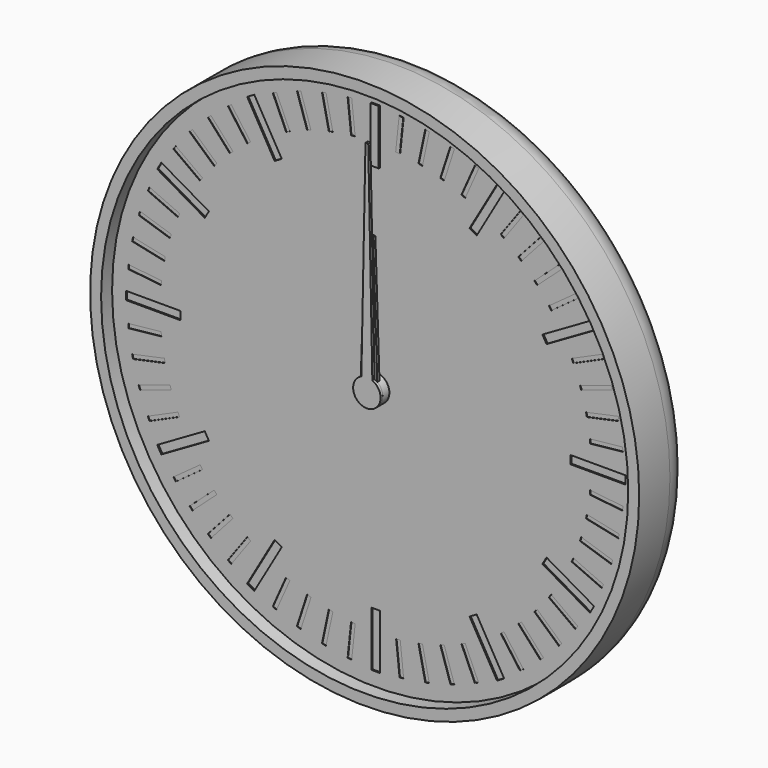
from build123d import *

# Parameters (mm, degrees)
F0_R      = 100
F1_DEPTH  = 24
F2_R      = 10
F3_T      = -4
F4_R      = 5
F4_R_2    = 3
F5_DEPTH  = 2
F6_DEPTH  = 19
F7_DEPTH  = 8
F9_DEPTH  = 4
F11_DEPTH = 4
F12_R     = 5
F12_R_2   = 3
F13_DEPTH = 2
F14_R     = 3
F15_DEPTH = 4
F17_DEPTH = 4
F18_R     = 3
F19_DEPTH = 2
F20_R     = 98
F20_R_2   = 5
F21_DEPTH = 1
F23_R     = 5
F23_R_2   = 3
F24_DEPTH = 2
F25_W     = 3
F25_H     = 20
F25_W_2   = 20
F25_H_2   = 3
F26_DEPTH = 0.5
F27_W     = 1.5
F27_H     = 12
F27_W_2   = 12
F27_H_2   = 1.5
F28_DEPTH = 0.2
F29_DEPTH = 1
F30_DEPTH = 0.4
F31_R     = 5
F31_R_2   = 3
F32_DEPTH = 5
F33_R     = 3
F34_DEPTH = 1
F36_DEPTH = 1


with BuildPart() as f1:
    # F0 (on Front) → F1 (new body)
    with BuildSketch(Plane.XZ):
        Circle(F0_R)
    extrude(amount=F1_DEPTH)

    # F2
    f2_edges = [f1.edges().sort_by_distance(p)[0] for p in [
        (-100, 0, 0),
    ]]
    fillet(f2_edges, radius=F2_R)

    # F3
    f3_openings = [f1.faces().sort_by_distance(p)[0] for p in [
        (0, -24, 0),
    ]]
    offset(amount=F3_T, openings=f3_openings)

    # F4 (on face) → F5 (join)
    with BuildSketch(Plane.XZ.offset(4)):
        Circle(F4_R)
        Circle(F4_R_2, mode=Mode.SUBTRACT)
        with Locations((40, 0)):
            Circle(F4_R)
        with Locations((40, 0)):
            Circle(F4_R_2, mode=Mode.SUBTRACT)
    extrude(amount=F5_DEPTH)


with BuildPart() as f6:
    # F6 (new): a face of the model
    f6_faces = [f1.part.faces().sort_by_distance(p)[0] for p in [
        (0, -4, 0),
    ]]
    extrude(f6_faces, amount=F6_DEPTH)

    # F8 (on face) → F9 (join)
    with BuildSketch(Plane.XZ.offset(6)):
        with BuildLine():
            ThreePointArc((9.2729637667, -1.3794085621), (9.3494561423, -0.6915886375), (9.375, 0))
            ThreePointArc((9.375, 0), (9.3494561423, 0.6915886375), (9.2729637667, 1.3794085621))
            ThreePointArc((9.2729637667, 1.3794085621), (8.9161548403, 2.8970343223), (8.3127812852, 4.3345463782))
            ThreePointArc((8.3127812852, 4.3345463782), (7.5845343223, 5.5104867402), (6.6911892658, 6.566476316))
            ThreePointArc((6.6911892658, 6.566476316), (5.5104867402, 7.5845343223), (4.1773988938, 8.3928519278))
            ThreePointArc((4.1773988938, 8.3928519278), (2.8970343223, 8.9161548403), (1.5536078905, 9.2453733036))
            ThreePointArc((1.5536078905, 9.2453733036), (0, 9.375), (-1.5536078905, 9.2453733036))
            ThreePointArc((-1.5536078905, 9.2453733036), (-2.8970343223, 8.9161548403), (-4.1773988938, 8.3928519278))
            ThreePointArc((-4.1773988938, 8.3928519278), (-5.5104867402, 7.5845343223), (-6.6911892658, 6.566476316))
            ThreePointArc((-6.6911892658, 6.566476316), (-7.5845343223, 5.5104867402), (-8.3127812852, 4.3345463782))
            ThreePointArc((-8.3127812852, 4.3345463782), (-8.9161548403, 2.8970343223), (-9.2729637667, 1.3794085621))
            ThreePointArc((-9.2729637667, 1.3794085621), (-9.375, 0), (-9.2729637667, -1.3794085621))
            ThreePointArc((-9.2729637667, -1.3794085621), (-8.9161548403, -2.8970343223), (-8.3127812852, -4.3345463782))
            ThreePointArc((-8.3127812852, -4.3345463782), (-7.5845343223, -5.5104867402), (-6.6911892658, -6.566476316))
            ThreePointArc((-6.6911892658, -6.566476316), (-5.5104867402, -7.5845343223), (-4.1773988938, -8.3928519278))
            ThreePointArc((-4.1773988938, -8.3928519278), (-2.8970343223, -8.9161548403), (-1.5536078905, -9.2453733036))
            ThreePointArc((-1.5536078905, -9.2453733036), (0, -9.375), (1.5536078905, -9.2453733036))
            ThreePointArc((1.5536078905, -9.2453733036), (2.8970343223, -8.9161548403), (4.1773988938, -8.3928519278))
            ThreePointArc((4.1773988938, -8.3928519278), (5.5104867402, -7.5845343223), (6.6911892658, -6.566476316))
            ThreePointArc((6.6911892658, -6.566476316), (7.5845343223, -5.5104867402), (8.3127812852, -4.3345463782))
            ThreePointArc((8.3127812852, -4.3345463782), (8.9161548403, -2.8970343223), (9.2729637667, -1.3794085621))
        make_face()
        with BuildLine():
            ThreePointArc((8.3127812852, 4.3345463782), (8.9161548403, 2.8970343223), (9.2729637667, 1.3794085621))
            Line((9.2729637667, 1.3794085621), (11.1823199426, 2.3946312492))
            Line((11.1823199426, 2.3946312492), (10.8182678729, 3.515068311))
            Line((10.8182678729, 3.515068311), (10.4542158031, 4.6355053728))
            Line((10.4542158031, 4.6355053728), (8.3127812852, 4.3345463782))
        make_face()
        with BuildLine():
            Line((11.1823199426, -2.3946312492), (9.2729637667, -1.3794085621))
            ThreePointArc((9.2729637667, -1.3794085621), (8.9161548403, -2.8970343223), (8.3127812852, -4.3345463782))
            Line((8.3127812852, -4.3345463782), (10.4542158031, -4.6355053728))
            Line((10.4542158031, -4.6355053728), (10.8182678729, -3.515068311))
            Line((10.8182678729, -3.515068311), (11.1823199426, -2.3946312492))
        make_face()
        with BuildLine():
            ThreePointArc((4.1773988938, 8.3928519278), (5.5104867402, 7.5845343223), (6.6911892658, 6.566476316))
            Line((6.6911892658, 6.566476316), (7.6391579371, 8.5101001246))
            Line((7.6391579371, 8.5101001246), (6.6860572448, 9.202568311))
            Line((6.6860572448, 9.202568311), (5.7329565525, 9.8950364974))
            Line((5.7329565525, 9.8950364974), (4.1773988938, 8.3928519278))
        make_face()
        with BuildLine():
            Line((7.6391579371, -8.5101001246), (6.6911892658, -6.566476316))
            ThreePointArc((6.6911892658, -6.566476316), (5.5104867402, -7.5845343223), (4.1773988938, -8.3928519278))
            Line((4.1773988938, -8.3928519278), (5.7329565525, -9.8950364974))
            Line((5.7329565525, -9.8950364974), (6.6860572448, -9.202568311))
            Line((6.6860572448, -9.202568311), (7.6391579371, -8.5101001246))
        make_face()
        with BuildLine():
            ThreePointArc((-1.5536078905, 9.2453733036), (0, 9.375), (1.5536078905, 9.2453733036))
            Line((1.5536078905, 9.2453733036), (1.1780972451, 11.375))
            Line((1.1780972451, 11.375), (0, 11.375))
            Line((0, 11.375), (-1.1780972451, 11.375))
            Line((-1.1780972451, 11.375), (-1.5536078905, 9.2453733036))
        make_face()
        with BuildLine():
            Line((1.1780972451, -11.375), (1.5536078905, -9.2453733036))
            ThreePointArc((1.5536078905, -9.2453733036), (0, -9.375), (-1.5536078905, -9.2453733036))
            Line((-1.5536078905, -9.2453733036), (-1.1780972451, -11.375))
            Line((-1.1780972451, -11.375), (0, -11.375))
            Line((0, -11.375), (1.1780972451, -11.375))
        make_face()
        with BuildLine():
            ThreePointArc((-6.6911892658, 6.566476316), (-5.5104867402, 7.5845343223), (-4.1773988938, 8.3928519278))
            Line((-4.1773988938, 8.3928519278), (-5.7329565525, 9.8950364974))
            Line((-5.7329565525, 9.8950364974), (-6.6860572448, 9.202568311))
            Line((-6.6860572448, 9.202568311), (-7.6391579371, 8.5101001246))
            Line((-7.6391579371, 8.5101001246), (-6.6911892658, 6.566476316))
        make_face()
        with BuildLine():
            Line((-5.7329565525, -9.8950364974), (-4.1773988938, -8.3928519278))
            ThreePointArc((-4.1773988938, -8.3928519278), (-5.5104867402, -7.5845343223), (-6.6911892658, -6.566476316))
            Line((-6.6911892658, -6.566476316), (-7.6391579371, -8.5101001246))
            Line((-7.6391579371, -8.5101001246), (-6.6860572448, -9.202568311))
            Line((-6.6860572448, -9.202568311), (-5.7329565525, -9.8950364974))
        make_face()
        with BuildLine():
            ThreePointArc((-9.2729637667, 1.3794085621), (-8.9161548403, 2.8970343223), (-8.3127812852, 4.3345463782))
            Line((-8.3127812852, 4.3345463782), (-10.4542158031, 4.6355053728))
            Line((-10.4542158031, 4.6355053728), (-10.8182678729, 3.515068311))
            Line((-10.8182678729, 3.515068311), (-11.1823199426, 2.3946312492))
            Line((-11.1823199426, 2.3946312492), (-9.2729637667, 1.3794085621))
        make_face()
        with BuildLine():
            Line((-10.4542158031, -4.6355053728), (-8.3127812852, -4.3345463782))
            ThreePointArc((-8.3127812852, -4.3345463782), (-8.9161548403, -2.8970343223), (-9.2729637667, -1.3794085621))
            Line((-9.2729637667, -1.3794085621), (-11.1823199426, -2.3946312492))
            Line((-11.1823199426, -2.3946312492), (-10.8182678729, -3.515068311))
            Line((-10.8182678729, -3.515068311), (-10.4542158031, -4.6355053728))
        make_face()
    extrude(amount=F9_DEPTH)

    # F35 (on face) → F36 (join)
    with BuildSketch(Plane.XZ.offset(23)):
        with BuildLine():
            ThreePointArc((-2, 4.582575695), (-2.7386127875, -4.1833001327), (5, 0))
            ThreePointArc((5, 0), (4.1833001327, 2.7386127875), (2, 4.582575695))
            ThreePointArc((2, 4.582575695), (0, 5), (-2, 4.582575695))
        make_face()
        with BuildLine():
            ThreePointArc((-2, 4.582575695), (0, 5), (2, 4.582575695))
            Line((2, 4.582575695), (0.5, 80))
            Line((0.5, 80), (0, 80))
            Line((0, 80), (-0.5, 80))
            Line((-0.5, 80), (-2, 4.582575695))
        make_face()
    extrude(amount=-F36_DEPTH)


with BuildPart() as f7:
    # F7 (new): a face of the model
    f7_faces = [f1.part.faces().sort_by_distance(p)[0] for p in [
        (40, -4, 0),
    ]]
    extrude(f7_faces, amount=F7_DEPTH)

    # F10 (on face) → F11 (join)
    with BuildSketch(Plane.XZ.offset(6)):
        with BuildLine():
            ThreePointArc((68.0829066802, -1.5381733945), (68.1144747006, -0.7693746225), (68.125, 0))
            ThreePointArc((68.125, 0), (68.1144747006, 0.7693746225), (68.0829066802, 1.5381733945))
            ThreePointArc((68.0829066802, 1.5381733945), (67.9709283072, 2.9398630294), (67.7890320221, 4.3342039956))
            ThreePointArc((67.7890320221, 4.3342039956), (67.5104012706, 5.8475163042), (67.1494235596, 7.3433252263))
            ThreePointArc((67.1494235596, 7.3433252263), (66.7484645208, 8.6911029668), (66.280643318, 10.0171558733))
            ThreePointArc((66.280643318, 10.0171558733), (65.6934659962, 11.4394680865), (65.0293803521, 12.8275385085))
            ThreePointArc((65.0293803521, 12.8275385085), (64.3569644814, 14.0625), (63.6236643925, 15.2623099717))
            ThreePointArc((63.6236643925, 15.2623099717), (62.7536029668, 16.5314602207), (61.815433119, 17.7511268046))
            ThreePointArc((61.815433119, 17.7511268046), (60.9009482166, 18.8192983038), (59.934217974, 19.8404278876))
            ThreePointArc((59.934217974, 19.8404278876), (58.8192983038, 20.9009482166), (57.6480467764, 21.8989056799))
            ThreePointArc((57.6480467764, 21.8989056799), (56.5314602207, 22.7536029668), (55.3735505752, 23.5514238999))
            ThreePointArc((55.3735505752, 23.5514238999), (54.0625, 24.3569644814), (52.709356105, 25.0895972944))
            ThreePointArc((52.709356105, 25.0895972944), (51.4394680865, 25.6934659962), (50.1409852457, 26.2331096755))
            ThreePointArc((50.1409852457, 26.2331096755), (48.6911029668, 26.7484645208), (47.2152055856, 27.1837531139))
            ThreePointArc((47.2152055856, 27.1837531139), (45.8475163042, 27.5104012706), (44.4652101991, 27.7682826779))
            ThreePointArc((44.4652101991, 27.7682826779), (42.9398630294, 27.9709283072), (41.4057159597, 28.0898484802))
            ThreePointArc((41.4057159597, 28.0898484802), (40, 28.125), (38.5942840403, 28.0898484802))
            ThreePointArc((38.5942840403, 28.0898484802), (37.0601369706, 27.9709283072), (35.5347898009, 27.7682826779))
            ThreePointArc((35.5347898009, 27.7682826779), (34.1524836958, 27.5104012706), (32.7847944144, 27.1837531139))
            ThreePointArc((32.7847944144, 27.1837531139), (31.3088970332, 26.7484645208), (29.8590147543, 26.2331096755))
            ThreePointArc((29.8590147543, 26.2331096755), (28.5605319135, 25.6934659962), (27.290643895, 25.0895972944))
            ThreePointArc((27.290643895, 25.0895972944), (25.9375, 24.3569644814), (24.6264494248, 23.5514238999))
            ThreePointArc((24.6264494248, 23.5514238999), (23.4685397793, 22.7536029668), (22.3519532236, 21.8989056799))
            ThreePointArc((22.3519532236, 21.8989056799), (21.1807016962, 20.9009482166), (20.065782026, 19.8404278876))
            ThreePointArc((20.065782026, 19.8404278876), (19.0990517834, 18.8192983038), (18.184566881, 17.7511268046))
            ThreePointArc((18.184566881, 17.7511268046), (17.2463970332, 16.5314602207), (16.3763356075, 15.2623099717))
            ThreePointArc((16.3763356075, 15.2623099717), (15.6430355186, 14.0625), (14.9706196479, 12.8275385085))
            ThreePointArc((14.9706196479, 12.8275385085), (14.3065340038, 11.4394680865), (13.719356682, 10.0171558733))
            ThreePointArc((13.719356682, 10.0171558733), (13.2515354792, 8.6911029668), (12.8505764404, 7.3433252263))
            ThreePointArc((12.8505764404, 7.3433252263), (12.4895987294, 5.8475163042), (12.2109679779, 4.3342039956))
            ThreePointArc((12.2109679779, 4.3342039956), (12.0290716928, 2.9398630294), (11.9170933198, 1.5381733945))
            ThreePointArc((11.9170933198, 1.5381733945), (11.875, 0), (11.9170933198, -1.5381733945))
            ThreePointArc((11.9170933198, -1.5381733945), (12.0290716928, -2.9398630294), (12.2109679779, -4.3342039956))
            ThreePointArc((12.2109679779, -4.3342039956), (12.4895987294, -5.8475163042), (12.8505764404, -7.3433252263))
            ThreePointArc((12.8505764404, -7.3433252263), (13.2515354792, -8.6911029668), (13.719356682, -10.0171558733))
            ThreePointArc((13.719356682, -10.0171558733), (14.3065340038, -11.4394680865), (14.9706196479, -12.8275385085))
            ThreePointArc((14.9706196479, -12.8275385085), (15.6430355186, -14.0625), (16.3763356075, -15.2623099717))
            ThreePointArc((16.3763356075, -15.2623099717), (17.2463970332, -16.5314602207), (18.184566881, -17.7511268046))
            ThreePointArc((18.184566881, -17.7511268046), (19.0990517834, -18.8192983038), (20.065782026, -19.8404278876))
            ThreePointArc((20.065782026, -19.8404278876), (21.1807016962, -20.9009482166), (22.3519532236, -21.8989056799))
            ThreePointArc((22.3519532236, -21.8989056799), (23.4685397793, -22.7536029668), (24.6264494248, -23.5514238999))
            ThreePointArc((24.6264494248, -23.5514238999), (25.9375, -24.3569644814), (27.290643895, -25.0895972944))
            ThreePointArc((27.290643895, -25.0895972944), (28.5605319135, -25.6934659962), (29.8590147543, -26.2331096755))
            ThreePointArc((29.8590147543, -26.2331096755), (31.3088970332, -26.7484645208), (32.7847944144, -27.1837531139))
            ThreePointArc((32.7847944144, -27.1837531139), (34.1524836958, -27.5104012706), (35.5347898009, -27.7682826779))
            ThreePointArc((35.5347898009, -27.7682826779), (37.0601369706, -27.9709283072), (38.5942840403, -28.0898484802))
            ThreePointArc((38.5942840403, -28.0898484802), (40, -28.125), (41.4057159597, -28.0898484802))
            ThreePointArc((41.4057159597, -28.0898484802), (42.9398630294, -27.9709283072), (44.4652101991, -27.7682826779))
            ThreePointArc((44.4652101991, -27.7682826779), (45.8475163042, -27.5104012706), (47.2152055856, -27.1837531139))
            ThreePointArc((47.2152055856, -27.1837531139), (48.6911029668, -26.7484645208), (50.1409852457, -26.2331096755))
            ThreePointArc((50.1409852457, -26.2331096755), (51.4394680865, -25.6934659962), (52.709356105, -25.0895972944))
            ThreePointArc((52.709356105, -25.0895972944), (54.0625, -24.3569644814), (55.3735505752, -23.5514238999))
            ThreePointArc((55.3735505752, -23.5514238999), (56.5314602207, -22.7536029668), (57.6480467764, -21.8989056799))
            ThreePointArc((57.6480467764, -21.8989056799), (58.8192983038, -20.9009482166), (59.934217974, -19.8404278876))
            ThreePointArc((59.934217974, -19.8404278876), (60.9009482166, -18.8192983038), (61.815433119, -17.7511268046))
            ThreePointArc((61.815433119, -17.7511268046), (62.7536029668, -16.5314602207), (63.6236643925, -15.2623099717))
            ThreePointArc((63.6236643925, -15.2623099717), (64.3569644814, -14.0625), (65.0293803521, -12.8275385085))
            ThreePointArc((65.0293803521, -12.8275385085), (65.6934659962, -11.4394680865), (66.280643318, -10.0171558733))
            ThreePointArc((66.280643318, -10.0171558733), (66.7484645208, -8.6911029668), (67.1494235596, -7.3433252263))
            ThreePointArc((67.1494235596, -7.3433252263), (67.5104012706, -5.8475163042), (67.7890320221, -4.3342039956))
            ThreePointArc((67.7890320221, -4.3342039956), (67.9709283072, -2.9398630294), (68.0829066802, -1.5381733945))
        make_face()
        with BuildLine():
            ThreePointArc((68.0829066802, 1.5381733945), (68.1144747006, 0.7693746225), (68.125, 0))
            ThreePointArc((68.125, 0), (68.1144747006, -0.7693746225), (68.0829066802, -1.5381733945))
            Line((68.0829066802, -1.5381733945), (70.125, -1.1780972451))
            Line((70.125, -1.1780972451), (70.125, 0))
            Line((70.125, 0), (70.125, 1.1780972451))
            Line((70.125, 1.1780972451), (68.0829066802, 1.5381733945))
        make_face()
        with BuildLine():
            ThreePointArc((67.1494235596, 7.3433252263), (67.5104012706, 5.8475163042), (67.7890320221, 4.3342039956))
            Line((67.7890320221, 4.3342039956), (69.7116366623, 5.1109866922))
            Line((69.7116366623, 5.1109866922), (69.4666964721, 6.2633396859))
            Line((69.4666964721, 6.2633396859), (69.2217562819, 7.4156926796))
            Line((69.2217562819, 7.4156926796), (67.1494235596, 7.3433252263))
        make_face()
        with BuildLine():
            Line((69.7116366623, -5.1109866922), (67.7890320221, -4.3342039956))
            ThreePointArc((67.7890320221, -4.3342039956), (67.5104012706, -5.8475163042), (67.1494235596, -7.3433252263))
            Line((67.1494235596, -7.3433252263), (69.2217562819, -7.4156926796))
            Line((69.2217562819, -7.4156926796), (69.4666964721, -6.2633396859))
            Line((69.4666964721, -6.2633396859), (69.7116366623, -5.1109866922))
        make_face()
        with BuildLine():
            ThreePointArc((65.0293803521, 12.8275385085), (65.6934659962, 11.4394680865), (66.280643318, 10.0171558733))
            Line((66.280643318, 10.0171558733), (67.9997322302, 11.1766959857))
            Line((67.9997322302, 11.1766959857), (67.5205569115, 12.2529413727))
            Line((67.5205569115, 12.2529413727), (67.0413815928, 13.3291867596))
            Line((67.0413815928, 13.3291867596), (65.0293803521, 12.8275385085))
        make_face()
        with BuildLine():
            Line((67.9997322302, -11.1766959857), (66.280643318, -10.0171558733))
            ThreePointArc((66.280643318, -10.0171558733), (65.6934659962, -11.4394680865), (65.0293803521, -12.8275385085))
            Line((65.0293803521, -12.8275385085), (67.0413815928, -13.3291867596))
            Line((67.0413815928, -13.3291867596), (67.5205569115, -12.2529413727))
            Line((67.5205569115, -12.2529413727), (67.9997322302, -11.1766959857))
        make_face()
        with BuildLine():
            ThreePointArc((61.815433119, 17.7511268046), (62.7536029668, 16.5314602207), (63.6236643925, 15.2623099717))
            Line((63.6236643925, 15.2623099717), (65.064105142, 16.753930033))
            Line((65.064105142, 16.753930033), (64.3716369555, 17.7070307253))
            Line((64.3716369555, 17.7070307253), (63.6791687691, 18.6601314176))
            Line((63.6791687691, 18.6601314176), (61.815433119, 17.7511268046))
        make_face()
        with BuildLine():
            Line((65.064105142, -16.753930033), (63.6236643925, -15.2623099717))
            ThreePointArc((63.6236643925, -15.2623099717), (62.7536029668, -16.5314602207), (61.815433119, -17.7511268046))
            Line((61.815433119, -17.7511268046), (63.6791687691, -18.6601314176))
            Line((63.6791687691, -18.6601314176), (64.3716369555, -17.7070307253))
            Line((64.3716369555, -17.7070307253), (65.064105142, -16.753930033))
        make_face()
        with BuildLine():
            ThreePointArc((57.6480467764, 21.8989056799), (58.8192983038, 20.9009482166), (59.934217974, 19.8404278876))
            Line((59.934217974, 19.8404278876), (61.0330563882, 21.5989369435))
            Line((61.0330563882, 21.5989369435), (60.1575595166, 22.3872378675))
            Line((60.1575595166, 22.3872378675), (59.282062645, 23.1755387915))
            Line((59.282062645, 23.1755387915), (57.6480467764, 21.8989056799))
        make_face()
        with BuildLine():
            Line((61.0330563882, -21.5989369435), (59.934217974, -19.8404278876))
            ThreePointArc((59.934217974, -19.8404278876), (58.8192983038, -20.9009482166), (57.6480467764, -21.8989056799))
            Line((57.6480467764, -21.8989056799), (59.282062645, -23.1755387915))
            Line((59.282062645, -23.1755387915), (60.1575595166, -22.3872378675))
            Line((60.1575595166, -22.3872378675), (61.0330563882, -21.5989369435))
        make_face()
        with BuildLine():
            ThreePointArc((52.709356105, 25.0895972944), (54.0625, 24.3569644814), (55.3735505752, 23.5514238999))
            Line((55.3735505752, 23.5514238999), (56.0827621424, 25.4999666665))
            Line((56.0827621424, 25.4999666665), (55.0625, 26.089015289))
            Line((55.0625, 26.089015289), (54.0422378576, 26.6780639116))
            Line((54.0422378576, 26.6780639116), (52.709356105, 25.0895972944))
        make_face()
        with BuildLine():
            Line((56.0827621424, -25.4999666665), (55.3735505752, -23.5514238999))
            ThreePointArc((55.3735505752, -23.5514238999), (54.0625, -24.3569644814), (52.709356105, -25.0895972944))
            Line((52.709356105, -25.0895972944), (54.0422378576, -26.6780639116))
            Line((54.0422378576, -26.6780639116), (55.0625, -26.089015289))
            Line((55.0625, -26.089015289), (56.0827621424, -25.4999666665))
        make_face()
        with BuildLine():
            ThreePointArc((47.2152055856, 27.1837531139), (48.6911029668, 26.7484645208), (50.1409852457, 26.2331096755))
            Line((50.1409852457, 26.2331096755), (50.4295740173, 28.2865254836))
            Line((50.4295740173, 28.2865254836), (49.3091369555, 28.6505775534))
            Line((49.3091369555, 28.6505775534), (48.1886998938, 29.0146296232))
            Line((48.1886998938, 29.0146296232), (47.2152055856, 27.1837531139))
        make_face()
        with BuildLine():
            Line((50.4295740173, -28.2865254836), (50.1409852457, -26.2331096755))
            ThreePointArc((50.1409852457, -26.2331096755), (48.6911029668, -26.7484645208), (47.2152055856, -27.1837531139))
            Line((47.2152055856, -27.1837531139), (48.1886998938, -29.0146296232))
            Line((48.1886998938, -29.0146296232), (49.3091369555, -28.6505775534))
            Line((49.3091369555, -28.6505775534), (50.4295740173, -28.2865254836))
        make_face()
        with BuildLine():
            ThreePointArc((41.4057159597, 28.0898484802), (42.9398630294, 27.9709283072), (44.4652101991, 27.7682826779))
            Line((44.4652101991, 27.7682826779), (44.3205634611, 29.8368274034))
            Line((44.3205634611, 29.8368274034), (43.1489199559, 29.959972098))
            Line((43.1489199559, 29.959972098), (41.9772764508, 30.0831167926))
            Line((41.9772764508, 30.0831167926), (41.4057159597, 28.0898484802))
        make_face()
        with BuildLine():
            Line((44.3205634611, -29.8368274034), (44.4652101991, -27.7682826779))
            ThreePointArc((44.4652101991, -27.7682826779), (42.9398630294, -27.9709283072), (41.4057159597, -28.0898484802))
            Line((41.4057159597, -28.0898484802), (41.9772764508, -30.0831167926))
            Line((41.9772764508, -30.0831167926), (43.1489199559, -29.959972098))
            Line((43.1489199559, -29.959972098), (44.3205634611, -29.8368274034))
        make_face()
        with BuildLine():
            ThreePointArc((35.5347898009, 27.7682826779), (37.0601369706, 27.9709283072), (38.5942840403, 28.0898484802))
            Line((38.5942840403, 28.0898484802), (38.0227235492, 30.0831167926))
            Line((38.0227235492, 30.0831167926), (36.8510800441, 29.959972098))
            Line((36.8510800441, 29.959972098), (35.6794365389, 29.8368274034))
            Line((35.6794365389, 29.8368274034), (35.5347898009, 27.7682826779))
        make_face()
        with BuildLine():
            Line((38.0227235492, -30.0831167926), (38.5942840403, -28.0898484802))
            ThreePointArc((38.5942840403, -28.0898484802), (37.0601369706, -27.9709283072), (35.5347898009, -27.7682826779))
            Line((35.5347898009, -27.7682826779), (35.6794365389, -29.8368274034))
            Line((35.6794365389, -29.8368274034), (36.8510800441, -29.959972098))
            Line((36.8510800441, -29.959972098), (38.0227235492, -30.0831167926))
        make_face()
        with BuildLine():
            ThreePointArc((29.8590147543, 26.2331096755), (31.3088970332, 26.7484645208), (32.7847944144, 27.1837531139))
            Line((32.7847944144, 27.1837531139), (31.8113001062, 29.0146296232))
            Line((31.8113001062, 29.0146296232), (30.6908630445, 28.6505775534))
            Line((30.6908630445, 28.6505775534), (29.5704259827, 28.2865254836))
            Line((29.5704259827, 28.2865254836), (29.8590147543, 26.2331096755))
        make_face()
        with BuildLine():
            Line((31.8113001062, -29.0146296232), (32.7847944144, -27.1837531139))
            ThreePointArc((32.7847944144, -27.1837531139), (31.3088970332, -26.7484645208), (29.8590147543, -26.2331096755))
            Line((29.8590147543, -26.2331096755), (29.5704259827, -28.2865254836))
            Line((29.5704259827, -28.2865254836), (30.6908630445, -28.6505775534))
            Line((30.6908630445, -28.6505775534), (31.8113001062, -29.0146296232))
        make_face()
        with BuildLine():
            ThreePointArc((24.6264494248, 23.5514238999), (25.9375, 24.3569644814), (27.290643895, 25.0895972944))
            Line((27.290643895, 25.0895972944), (25.9577621424, 26.6780639116))
            Line((25.9577621424, 26.6780639116), (24.9375, 26.089015289))
            Line((24.9375, 26.089015289), (23.9172378576, 25.4999666665))
            Line((23.9172378576, 25.4999666665), (24.6264494248, 23.5514238999))
        make_face()
        with BuildLine():
            Line((25.9577621424, -26.6780639116), (27.290643895, -25.0895972944))
            ThreePointArc((27.290643895, -25.0895972944), (25.9375, -24.3569644814), (24.6264494248, -23.5514238999))
            Line((24.6264494248, -23.5514238999), (23.9172378576, -25.4999666665))
            Line((23.9172378576, -25.4999666665), (24.9375, -26.089015289))
            Line((24.9375, -26.089015289), (25.9577621424, -26.6780639116))
        make_face()
        with BuildLine():
            ThreePointArc((20.065782026, 19.8404278876), (21.1807016962, 20.9009482166), (22.3519532236, 21.8989056799))
            Line((22.3519532236, 21.8989056799), (20.717937355, 23.1755387915))
            Line((20.717937355, 23.1755387915), (19.8424404834, 22.3872378675))
            Line((19.8424404834, 22.3872378675), (18.9669436118, 21.5989369435))
            Line((18.9669436118, 21.5989369435), (20.065782026, 19.8404278876))
        make_face()
        with BuildLine():
            Line((20.717937355, -23.1755387915), (22.3519532236, -21.8989056799))
            ThreePointArc((22.3519532236, -21.8989056799), (21.1807016962, -20.9009482166), (20.065782026, -19.8404278876))
            Line((20.065782026, -19.8404278876), (18.9669436118, -21.5989369435))
            Line((18.9669436118, -21.5989369435), (19.8424404834, -22.3872378675))
            Line((19.8424404834, -22.3872378675), (20.717937355, -23.1755387915))
        make_face()
        with BuildLine():
            ThreePointArc((16.3763356075, 15.2623099717), (17.2463970332, 16.5314602207), (18.184566881, 17.7511268046))
            Line((18.184566881, 17.7511268046), (16.3208312309, 18.6601314176))
            Line((16.3208312309, 18.6601314176), (15.6283630445, 17.7070307253))
            Line((15.6283630445, 17.7070307253), (14.935894858, 16.753930033))
            Line((14.935894858, 16.753930033), (16.3763356075, 15.2623099717))
        make_face()
        with BuildLine():
            Line((16.3208312309, -18.6601314176), (18.184566881, -17.7511268046))
            ThreePointArc((18.184566881, -17.7511268046), (17.2463970332, -16.5314602207), (16.3763356075, -15.2623099717))
            Line((16.3763356075, -15.2623099717), (14.935894858, -16.753930033))
            Line((14.935894858, -16.753930033), (15.6283630445, -17.7070307253))
            Line((15.6283630445, -17.7070307253), (16.3208312309, -18.6601314176))
        make_face()
        with BuildLine():
            ThreePointArc((13.719356682, 10.0171558733), (14.3065340038, 11.4394680865), (14.9706196479, 12.8275385085))
            Line((14.9706196479, 12.8275385085), (12.9586184072, 13.3291867596))
            Line((12.9586184072, 13.3291867596), (12.4794430885, 12.2529413727))
            Line((12.4794430885, 12.2529413727), (12.0002677698, 11.1766959857))
            Line((12.0002677698, 11.1766959857), (13.719356682, 10.0171558733))
        make_face()
        with BuildLine():
            Line((12.9586184072, -13.3291867596), (14.9706196479, -12.8275385085))
            ThreePointArc((14.9706196479, -12.8275385085), (14.3065340038, -11.4394680865), (13.719356682, -10.0171558733))
            Line((13.719356682, -10.0171558733), (12.0002677698, -11.1766959857))
            Line((12.0002677698, -11.1766959857), (12.4794430885, -12.2529413727))
            Line((12.4794430885, -12.2529413727), (12.9586184072, -13.3291867596))
        make_face()
        with BuildLine():
            ThreePointArc((12.2109679779, 4.3342039956), (12.4895987294, 5.8475163042), (12.8505764404, 7.3433252263))
            Line((12.8505764404, 7.3433252263), (10.7782437181, 7.4156926796))
            Line((10.7782437181, 7.4156926796), (10.5333035279, 6.2633396859))
            Line((10.5333035279, 6.2633396859), (10.2883633377, 5.1109866922))
            Line((10.2883633377, 5.1109866922), (12.2109679779, 4.3342039956))
        make_face()
        with BuildLine():
            Line((10.7782437181, -7.4156926796), (12.8505764404, -7.3433252263))
            ThreePointArc((12.8505764404, -7.3433252263), (12.4895987294, -5.8475163042), (12.2109679779, -4.3342039956))
            Line((12.2109679779, -4.3342039956), (10.2883633377, -5.1109866922))
            Line((10.2883633377, -5.1109866922), (10.5333035279, -6.2633396859))
            Line((10.5333035279, -6.2633396859), (10.7782437181, -7.4156926796))
        make_face()
        with BuildLine():
            ThreePointArc((11.9170933198, -1.5381733945), (11.875, 0), (11.9170933198, 1.5381733945))
            Line((11.9170933198, 1.5381733945), (9.875, 1.1780972451))
            Line((9.875, 1.1780972451), (9.875, 0))
            Line((9.875, 0), (9.875, -1.1780972451))
            Line((9.875, -1.1780972451), (11.9170933198, -1.5381733945))
        make_face()
    extrude(amount=F11_DEPTH)

    # F16 (on face) → F17 (join)
    with BuildSketch(Plane.XZ.offset(12)):
        with BuildLine():
            ThreePointArc((47.4288750323, -1.0304444454), (47.4821976298, -0.5164480894), (47.5, 0))
            ThreePointArc((47.5, 0), (47.4821976298, 0.5164480894), (47.4288750323, 1.0304444454))
            ThreePointArc((47.4288750323, 1.0304444454), (47.1329238722, 2.3176274578), (46.6157661985, 3.532936117))
            ThreePointArc((46.6157661985, 3.532936117), (46.0676274578, 4.4083893922), (45.4044061018, 5.2002302532))
            ThreePointArc((45.4044061018, 5.2002302532), (44.4083893922, 6.0676274578), (43.2756595386, 6.7468551628))
            ThreePointArc((43.2756595386, 6.7468551628), (42.3176274578, 7.1329238722), (41.3156377295, 7.3837048536))
            ThreePointArc((41.3156377295, 7.3837048536), (40, 7.5), (38.6843622705, 7.3837048536))
            ThreePointArc((38.6843622705, 7.3837048536), (37.6823725422, 7.1329238722), (36.7243404614, 6.7468551628))
            ThreePointArc((36.7243404614, 6.7468551628), (35.5916106078, 6.0676274578), (34.5955938982, 5.2002302532))
            ThreePointArc((34.5955938982, 5.2002302532), (33.9323725422, 4.4083893922), (33.3842338015, 3.532936117))
            ThreePointArc((33.3842338015, 3.532936117), (32.8670761278, 2.3176274578), (32.5711249677, 1.0304444454))
            ThreePointArc((32.5711249677, 1.0304444454), (32.5, 0), (32.5711249677, -1.0304444454))
            ThreePointArc((32.5711249677, -1.0304444454), (32.8670761278, -2.3176274578), (33.3842338015, -3.532936117))
            ThreePointArc((33.3842338015, -3.532936117), (33.9323725422, -4.4083893922), (34.5955938982, -5.2002302532))
            ThreePointArc((34.5955938982, -5.2002302532), (35.5916106078, -6.0676274578), (36.7243404614, -6.7468551628))
            ThreePointArc((36.7243404614, -6.7468551628), (37.6823725422, -7.1329238722), (38.6843622705, -7.3837048536))
            ThreePointArc((38.6843622705, -7.3837048536), (40, -7.5), (41.3156377295, -7.3837048536))
            ThreePointArc((41.3156377295, -7.3837048536), (42.3176274578, -7.1329238722), (43.2756595386, -6.7468551628))
            ThreePointArc((43.2756595386, -6.7468551628), (44.4083893922, -6.0676274578), (45.4044061018, -5.2002302532))
            ThreePointArc((45.4044061018, -5.2002302532), (46.0676274578, -4.4083893922), (46.6157661985, -3.532936117))
            ThreePointArc((46.6157661985, -3.532936117), (47.1329238722, -2.3176274578), (47.4288750323, -1.0304444454))
        make_face()
        with BuildLine():
            ThreePointArc((46.6157661985, 3.532936117), (47.1329238722, 2.3176274578), (47.4288750323, 1.0304444454))
            Line((47.4288750323, 1.0304444454), (49.3262785606, 2.0393117971))
            Line((49.3262785606, 2.0393117971), (48.743795249, 3.832011096))
            Line((48.743795249, 3.832011096), (46.6157661985, 3.532936117))
        make_face()
        with BuildLine():
            Line((49.3262785606, -2.0393117971), (47.4288750323, -1.0304444454))
            ThreePointArc((47.4288750323, -1.0304444454), (47.1329238722, -2.3176274578), (46.6157661985, -3.532936117))
            Line((46.6157661985, -3.532936117), (48.743795249, -3.832011096))
            Line((48.743795249, -3.832011096), (49.3262785606, -2.0393117971))
        make_face()
        with BuildLine():
            ThreePointArc((43.2756595386, 6.7468551628), (44.4083893922, 6.0676274578), (45.4044061018, 5.2002302532))
            Line((45.4044061018, 5.2002302532), (46.3464404506, 7.1316868974))
            Line((46.3464404506, 7.1316868974), (44.8214793429, 8.2396359957))
            Line((44.8214793429, 8.2396359957), (43.2756595386, 6.7468551628))
        make_face()
        with BuildLine():
            Line((46.3464404506, -7.1316868974), (45.4044061018, -5.2002302532))
            ThreePointArc((45.4044061018, -5.2002302532), (44.4083893922, -6.0676274578), (43.2756595386, -6.7468551628))
            Line((43.2756595386, -6.7468551628), (44.8214793429, -8.2396359957))
            Line((44.8214793429, -8.2396359957), (46.3464404506, -7.1316868974))
        make_face()
        with BuildLine():
            ThreePointArc((38.6843622705, 7.3837048536), (40, 7.5), (41.3156377295, 7.3837048536))
            Line((41.3156377295, 7.3837048536), (40.9424777961, 9.5))
            Line((40.9424777961, 9.5), (39.0575222039, 9.5))
            Line((39.0575222039, 9.5), (38.6843622705, 7.3837048536))
        make_face()
        with BuildLine():
            Line((40.9424777961, -9.5), (41.3156377295, -7.3837048536))
            ThreePointArc((41.3156377295, -7.3837048536), (40, -7.5), (38.6843622705, -7.3837048536))
            Line((38.6843622705, -7.3837048536), (39.0575222039, -9.5))
            Line((39.0575222039, -9.5), (40.9424777961, -9.5))
        make_face()
        with BuildLine():
            ThreePointArc((34.5955938982, 5.2002302532), (35.5916106078, 6.0676274578), (36.7243404614, 6.7468551628))
            Line((36.7243404614, 6.7468551628), (35.1785206571, 8.2396359957))
            Line((35.1785206571, 8.2396359957), (33.6535595494, 7.1316868974))
            Line((33.6535595494, 7.1316868974), (34.5955938982, 5.2002302532))
        make_face()
        with BuildLine():
            Line((35.1785206571, -8.2396359957), (36.7243404614, -6.7468551628))
            ThreePointArc((36.7243404614, -6.7468551628), (35.5916106078, -6.0676274578), (34.5955938982, -5.2002302532))
            Line((34.5955938982, -5.2002302532), (33.6535595494, -7.1316868974))
            Line((33.6535595494, -7.1316868974), (35.1785206571, -8.2396359957))
        make_face()
        with BuildLine():
            ThreePointArc((32.5711249677, 1.0304444454), (32.8670761278, 2.3176274578), (33.3842338015, 3.532936117))
            Line((33.3842338015, 3.532936117), (31.256204751, 3.832011096))
            Line((31.256204751, 3.832011096), (30.6737214394, 2.0393117971))
            Line((30.6737214394, 2.0393117971), (32.5711249677, 1.0304444454))
        make_face()
        with BuildLine():
            Line((31.256204751, -3.832011096), (33.3842338015, -3.532936117))
            ThreePointArc((33.3842338015, -3.532936117), (32.8670761278, -2.3176274578), (32.5711249677, -1.0304444454))
            Line((32.5711249677, -1.0304444454), (30.6737214394, -2.0393117971))
            Line((30.6737214394, -2.0393117971), (31.256204751, -3.832011096))
        make_face()
    extrude(amount=F17_DEPTH)

    # F18 (on face) → F19 (join)
    with BuildSketch(Plane.XZ.offset(16)):
        with Locations((40, 0)):
            Circle(F18_R)
    extrude(amount=F19_DEPTH)


with BuildPart() as f13:
    # F12 (on face) → F13 (new body)
    with BuildSketch(Plane.XZ.offset(10)):
        Circle(F12_R)
        Circle(F12_R_2, mode=Mode.SUBTRACT)
    extrude(amount=F13_DEPTH)

    # F14 (on face) → F15 (join)
    with BuildSketch(Plane.XZ.offset(12)):
        with BuildLine():
            ThreePointArc((29.9718156995, -1.3001014101), (29.9929530972, -0.6502034357), (30, 0))
            ThreePointArc((30, 0), (29.9929530972, 0.6502034357), (29.9718156995, 1.3001014101))
            ThreePointArc((29.9718156995, 1.3001014101), (29.907520012, 2.3537728718), (29.8061935814, 3.4045299509))
            ThreePointArc((29.8061935814, 3.4045299509), (29.6306502179, 4.6930339512), (29.3994322443, 5.9727199596))
            ThreePointArc((29.3994322443, 5.9727199596), (29.1710976119, 7.0033609157), (28.9066440563, 8.0253304855))
            ThreePointArc((28.9066440563, 8.0253304855), (28.5316954889, 9.2705098312), (28.1031371961, 10.4982703213))
            ThreePointArc((28.1031371961, 10.4982703213), (27.7163859753, 11.480502971), (27.2953170189, 12.448520749))
            ThreePointArc((27.2953170189, 12.448520749), (26.7301957257, 13.6197149922), (26.1148496411, 14.765318426))
            ThreePointArc((26.1148496411, 14.765318426), (25.5792049306, 15.6749569415), (25.0118886885, 16.5651871174))
            ThreePointArc((25.0118886885, 16.5651871174), (24.2705098312, 17.6335575688), (23.4835278178, 18.6687953878))
            ThreePointArc((23.4835278178, 18.6687953878), (22.812178968, 19.4834414499), (22.1125846489, 20.2739636023))
            ThreePointArc((22.1125846489, 20.2739636023), (21.2132034356, 21.2132034356), (20.2739636023, 22.1125846489))
            ThreePointArc((20.2739636023, 22.1125846489), (19.4834414499, 22.812178968), (18.6687953878, 23.4835278178))
            ThreePointArc((18.6687953878, 23.4835278178), (17.6335575688, 24.2705098312), (16.5651871174, 25.0118886885))
            ThreePointArc((16.5651871174, 25.0118886885), (15.6749569415, 25.5792049306), (14.765318426, 26.1148496411))
            ThreePointArc((14.765318426, 26.1148496411), (13.6197149922, 26.7301957257), (12.448520749, 27.2953170189))
            ThreePointArc((12.448520749, 27.2953170189), (11.480502971, 27.7163859753), (10.4982703213, 28.1031371961))
            ThreePointArc((10.4982703213, 28.1031371961), (9.2705098312, 28.5316954889), (8.0253304855, 28.9066440563))
            ThreePointArc((8.0253304855, 28.9066440563), (7.0033609157, 29.1710976119), (5.9727199596, 29.3994322443))
            ThreePointArc((5.9727199596, 29.3994322443), (4.6930339512, 29.6306502179), (3.4045299509, 29.8061935814))
            ThreePointArc((3.4045299509, 29.8061935814), (2.3537728718, 29.907520012), (1.3001014101, 29.9718156995))
            ThreePointArc((1.3001014101, 29.9718156995), (0, 30), (-1.3001014101, 29.9718156995))
            ThreePointArc((-1.3001014101, 29.9718156995), (-2.3537728718, 29.907520012), (-3.4045299509, 29.8061935814))
            ThreePointArc((-3.4045299509, 29.8061935814), (-4.6930339512, 29.6306502179), (-5.9727199596, 29.3994322443))
            ThreePointArc((-5.9727199596, 29.3994322443), (-7.0033609157, 29.1710976119), (-8.0253304855, 28.9066440563))
            ThreePointArc((-8.0253304855, 28.9066440563), (-9.2705098312, 28.5316954889), (-10.4982703213, 28.1031371961))
            ThreePointArc((-10.4982703213, 28.1031371961), (-11.480502971, 27.7163859753), (-12.448520749, 27.2953170189))
            ThreePointArc((-12.448520749, 27.2953170189), (-13.6197149922, 26.7301957257), (-14.765318426, 26.1148496411))
            ThreePointArc((-14.765318426, 26.1148496411), (-15.6749569415, 25.5792049306), (-16.5651871174, 25.0118886885))
            ThreePointArc((-16.5651871174, 25.0118886885), (-17.6335575688, 24.2705098312), (-18.6687953878, 23.4835278178))
            ThreePointArc((-18.6687953878, 23.4835278178), (-19.4834414499, 22.812178968), (-20.2739636023, 22.1125846489))
            ThreePointArc((-20.2739636023, 22.1125846489), (-21.2132034356, 21.2132034356), (-22.1125846489, 20.2739636023))
            ThreePointArc((-22.1125846489, 20.2739636023), (-22.812178968, 19.4834414499), (-23.4835278178, 18.6687953878))
            ThreePointArc((-23.4835278178, 18.6687953878), (-24.2705098312, 17.6335575688), (-25.0118886885, 16.5651871174))
            ThreePointArc((-25.0118886885, 16.5651871174), (-25.5792049306, 15.6749569415), (-26.1148496411, 14.765318426))
            ThreePointArc((-26.1148496411, 14.765318426), (-26.7301957257, 13.6197149922), (-27.2953170189, 12.448520749))
            ThreePointArc((-27.2953170189, 12.448520749), (-27.7163859753, 11.480502971), (-28.1031371961, 10.4982703213))
            ThreePointArc((-28.1031371961, 10.4982703213), (-28.5316954889, 9.2705098312), (-28.9066440563, 8.0253304855))
            ThreePointArc((-28.9066440563, 8.0253304855), (-29.1710976119, 7.0033609157), (-29.3994322443, 5.9727199596))
            ThreePointArc((-29.3994322443, 5.9727199596), (-29.6306502179, 4.6930339512), (-29.8061935814, 3.4045299509))
            ThreePointArc((-29.8061935814, 3.4045299509), (-29.907520012, 2.3537728718), (-29.9718156995, 1.3001014101))
            ThreePointArc((-29.9718156995, 1.3001014101), (-30, 0), (-29.9718156995, -1.3001014101))
            ThreePointArc((-29.9718156995, -1.3001014101), (-29.907520012, -2.3537728718), (-29.8061935814, -3.4045299509))
            ThreePointArc((-29.8061935814, -3.4045299509), (-29.6306502179, -4.6930339512), (-29.3994322443, -5.9727199596))
            ThreePointArc((-29.3994322443, -5.9727199596), (-29.1710976119, -7.0033609157), (-28.9066440563, -8.0253304855))
            ThreePointArc((-28.9066440563, -8.0253304855), (-28.5316954889, -9.2705098312), (-28.1031371961, -10.4982703213))
            ThreePointArc((-28.1031371961, -10.4982703213), (-27.7163859753, -11.480502971), (-27.2953170189, -12.448520749))
            ThreePointArc((-27.2953170189, -12.448520749), (-26.7301957257, -13.6197149922), (-26.1148496411, -14.765318426))
            ThreePointArc((-26.1148496411, -14.765318426), (-25.5792049306, -15.6749569415), (-25.0118886885, -16.5651871174))
            ThreePointArc((-25.0118886885, -16.5651871174), (-24.2705098312, -17.6335575688), (-23.4835278178, -18.6687953878))
            ThreePointArc((-23.4835278178, -18.6687953878), (-22.812178968, -19.4834414499), (-22.1125846489, -20.2739636023))
            ThreePointArc((-22.1125846489, -20.2739636023), (-21.2132034356, -21.2132034356), (-20.2739636023, -22.1125846489))
            ThreePointArc((-20.2739636023, -22.1125846489), (-19.4834414499, -22.812178968), (-18.6687953878, -23.4835278178))
            ThreePointArc((-18.6687953878, -23.4835278178), (-17.6335575688, -24.2705098312), (-16.5651871174, -25.0118886885))
            ThreePointArc((-16.5651871174, -25.0118886885), (-15.6749569415, -25.5792049306), (-14.765318426, -26.1148496411))
            ThreePointArc((-14.765318426, -26.1148496411), (-13.6197149922, -26.7301957257), (-12.448520749, -27.2953170189))
            ThreePointArc((-12.448520749, -27.2953170189), (-11.480502971, -27.7163859753), (-10.4982703213, -28.1031371961))
            ThreePointArc((-10.4982703213, -28.1031371961), (-9.2705098312, -28.5316954889), (-8.0253304855, -28.9066440563))
            ThreePointArc((-8.0253304855, -28.9066440563), (-7.0033609157, -29.1710976119), (-5.9727199596, -29.3994322443))
            ThreePointArc((-5.9727199596, -29.3994322443), (-4.6930339512, -29.6306502179), (-3.4045299509, -29.8061935814))
            ThreePointArc((-3.4045299509, -29.8061935814), (-2.3537728718, -29.907520012), (-1.3001014101, -29.9718156995))
            ThreePointArc((-1.3001014101, -29.9718156995), (0, -30), (1.3001014101, -29.9718156995))
            ThreePointArc((1.3001014101, -29.9718156995), (2.3537728718, -29.907520012), (3.4045299509, -29.8061935814))
            ThreePointArc((3.4045299509, -29.8061935814), (4.6930339512, -29.6306502179), (5.9727199596, -29.3994322443))
            ThreePointArc((5.9727199596, -29.3994322443), (7.0033609157, -29.1710976119), (8.0253304855, -28.9066440563))
            ThreePointArc((8.0253304855, -28.9066440563), (9.2705098312, -28.5316954889), (10.4982703213, -28.1031371961))
            ThreePointArc((10.4982703213, -28.1031371961), (11.480502971, -27.7163859753), (12.448520749, -27.2953170189))
            ThreePointArc((12.448520749, -27.2953170189), (13.6197149922, -26.7301957257), (14.765318426, -26.1148496411))
            ThreePointArc((14.765318426, -26.1148496411), (15.6749569415, -25.5792049306), (16.5651871174, -25.0118886885))
            ThreePointArc((16.5651871174, -25.0118886885), (17.6335575688, -24.2705098312), (18.6687953878, -23.4835278178))
            ThreePointArc((18.6687953878, -23.4835278178), (19.4834414499, -22.812178968), (20.2739636023, -22.1125846489))
            ThreePointArc((20.2739636023, -22.1125846489), (21.2132034356, -21.2132034356), (22.1125846489, -20.2739636023))
            ThreePointArc((22.1125846489, -20.2739636023), (22.812178968, -19.4834414499), (23.4835278178, -18.6687953878))
            ThreePointArc((23.4835278178, -18.6687953878), (24.2705098312, -17.6335575688), (25.0118886885, -16.5651871174))
            ThreePointArc((25.0118886885, -16.5651871174), (25.5792049306, -15.6749569415), (26.1148496411, -14.765318426))
            ThreePointArc((26.1148496411, -14.765318426), (26.7301957257, -13.6197149922), (27.2953170189, -12.448520749))
            ThreePointArc((27.2953170189, -12.448520749), (27.7163859753, -11.480502971), (28.1031371961, -10.4982703213))
            ThreePointArc((28.1031371961, -10.4982703213), (28.5316954889, -9.2705098312), (28.9066440563, -8.0253304855))
            ThreePointArc((28.9066440563, -8.0253304855), (29.1710976119, -7.0033609157), (29.3994322443, -5.9727199596))
            ThreePointArc((29.3994322443, -5.9727199596), (29.6306502179, -4.6930339512), (29.8061935814, -3.4045299509))
            ThreePointArc((29.8061935814, -3.4045299509), (29.907520012, -2.3537728718), (29.9718156995, -1.3001014101))
        make_face()
        Circle(F14_R, mode=Mode.SUBTRACT)
        with BuildLine():
            ThreePointArc((29.9718156995, 1.3001014101), (29.9929530972, 0.6502034357), (30, 0))
            ThreePointArc((30, 0), (29.9929530972, -0.6502034357), (29.9718156995, -1.3001014101))
            Line((29.9718156995, -1.3001014101), (32, -0.9424777961))
            Line((32, -0.9424777961), (32, 0))
            Line((32, 0), (32, 0.9424777961))
            Line((32, 0.9424777961), (29.9718156995, 1.3001014101))
        make_face()
        with BuildLine():
            ThreePointArc((29.3994322443, 5.9727199596), (29.6306502179, 4.6930339512), (29.8061935814, 3.4045299509))
            Line((29.8061935814, 3.4045299509), (31.7534629089, 4.0750285508))
            Line((31.7534629089, 4.0750285508), (31.606026899, 5.0059028813))
            Line((31.606026899, 5.0059028813), (31.4585908892, 5.9367772117))
            Line((31.4585908892, 5.9367772117), (29.3994322443, 5.9727199596))
        make_face()
        with BuildLine():
            Line((31.7534629089, -4.0750285508), (29.8061935814, -3.4045299509))
            ThreePointArc((29.8061935814, -3.4045299509), (29.6306502179, -4.6930339512), (29.3994322443, -5.9727199596))
            Line((29.3994322443, -5.9727199596), (31.4585908892, -5.9367772117))
            Line((31.4585908892, -5.9367772117), (31.606026899, -5.0059028813))
            Line((31.606026899, -5.0059028813), (31.7534629089, -4.0750285508))
        make_face()
        with BuildLine():
            ThreePointArc((28.1031371961, 10.4982703213), (28.5316954889, 9.2705098312), (28.9066440563, 8.0253304855))
            Line((28.9066440563, 8.0253304855), (30.7250501773, 8.9921941706))
            Line((30.7250501773, 8.9921941706), (30.4338085214, 9.88854382))
            Line((30.4338085214, 9.88854382), (30.1425668656, 10.7848934694))
            Line((30.1425668656, 10.7848934694), (28.1031371961, 10.4982703213))
        make_face()
        with BuildLine():
            Line((30.7250501773, -8.9921941706), (28.9066440563, -8.0253304855))
            ThreePointArc((28.9066440563, -8.0253304855), (28.5316954889, -9.2705098312), (28.1031371961, -10.4982703213))
            Line((28.1031371961, -10.4982703213), (30.1425668656, -10.7848934694))
            Line((30.1425668656, -10.7848934694), (30.4338085214, -9.88854382))
            Line((30.4338085214, -9.88854382), (30.7250501773, -8.9921941706))
        make_face()
        with BuildLine():
            ThreePointArc((26.1148496411, 14.765318426), (26.7301957257, 13.6197149922), (27.2953170189, 12.448520749))
            Line((27.2953170189, 12.448520749), (28.9400847397, 13.6879421265))
            Line((28.9400847397, 13.6879421265), (28.512208774, 14.5276959917))
            Line((28.512208774, 14.5276959917), (28.0843328084, 15.3674498569))
            Line((28.0843328084, 15.3674498569), (26.1148496411, 14.765318426))
        make_face()
        with BuildLine():
            Line((28.9400847397, -13.6879421265), (27.2953170189, -12.448520749))
            ThreePointArc((27.2953170189, -12.448520749), (26.7301957257, -13.6197149922), (26.1148496411, -14.765318426))
            Line((26.1148496411, -14.765318426), (28.0843328084, -15.3674498569))
            Line((28.0843328084, -15.3674498569), (28.512208774, -14.5276959917))
            Line((28.512208774, -14.5276959917), (28.9400847397, -13.6879421265))
        make_face()
        with BuildLine():
            ThreePointArc((23.4835278178, 18.6687953878), (24.2705098312, 17.6335575688), (25.0118886885, 16.5651871174))
            Line((25.0118886885, 16.5651871174), (26.4425183691, 18.0466475195))
            Line((26.4425183691, 18.0466475195), (25.88854382, 18.8091280734))
            Line((25.88854382, 18.8091280734), (25.3345692709, 19.5716086272))
            Line((25.3345692709, 19.5716086272), (23.4835278178, 18.6687953878))
        make_face()
        with BuildLine():
            Line((26.4425183691, -18.0466475195), (25.0118886885, -16.5651871174))
            ThreePointArc((25.0118886885, -16.5651871174), (24.2705098312, -17.6335575688), (23.4835278178, -18.6687953878))
            Line((23.4835278178, -18.6687953878), (25.3345692709, -19.5716086272))
            Line((25.3345692709, -19.5716086272), (25.88854382, -18.8091280734))
            Line((25.88854382, -18.8091280734), (26.4425183691, -18.0466475195))
        make_face()
        with BuildLine():
            ThreePointArc((20.2739636023, 22.1125846489), (21.2132034356, 21.2132034356), (22.1125846489, 20.2739636023))
            Line((22.1125846489, 20.2739636023), (23.2938494387, 21.9609845572))
            Line((23.2938494387, 21.9609845572), (22.627416998, 22.627416998))
            Line((22.627416998, 22.627416998), (21.9609845572, 23.2938494387))
            Line((21.9609845572, 23.2938494387), (20.2739636023, 22.1125846489))
        make_face()
        with BuildLine():
            Line((23.2938494387, -21.9609845572), (22.1125846489, -20.2739636023))
            ThreePointArc((22.1125846489, -20.2739636023), (21.2132034356, -21.2132034356), (20.2739636023, -22.1125846489))
            Line((20.2739636023, -22.1125846489), (21.9609845572, -23.2938494387))
            Line((21.9609845572, -23.2938494387), (22.627416998, -22.627416998))
            Line((22.627416998, -22.627416998), (23.2938494387, -21.9609845572))
        make_face()
        with BuildLine():
            ThreePointArc((16.5651871174, 25.0118886885), (17.6335575688, 24.2705098312), (18.6687953878, 23.4835278178))
            Line((18.6687953878, 23.4835278178), (19.5716086272, 25.3345692709))
            Line((19.5716086272, 25.3345692709), (18.8091280734, 25.88854382))
            Line((18.8091280734, 25.88854382), (18.0466475195, 26.4425183691))
            Line((18.0466475195, 26.4425183691), (16.5651871174, 25.0118886885))
        make_face()
        with BuildLine():
            Line((19.5716086272, -25.3345692709), (18.6687953878, -23.4835278178))
            ThreePointArc((18.6687953878, -23.4835278178), (17.6335575688, -24.2705098312), (16.5651871174, -25.0118886885))
            Line((16.5651871174, -25.0118886885), (18.0466475195, -26.4425183691))
            Line((18.0466475195, -26.4425183691), (18.8091280734, -25.88854382))
            Line((18.8091280734, -25.88854382), (19.5716086272, -25.3345692709))
        make_face()
        with BuildLine():
            ThreePointArc((12.448520749, 27.2953170189), (13.6197149922, 26.7301957257), (14.765318426, 26.1148496411))
            Line((14.765318426, 26.1148496411), (15.3674498569, 28.0843328084))
            Line((15.3674498569, 28.0843328084), (14.5276959917, 28.512208774))
            Line((14.5276959917, 28.512208774), (13.6879421265, 28.9400847397))
            Line((13.6879421265, 28.9400847397), (12.448520749, 27.2953170189))
        make_face()
        with BuildLine():
            Line((15.3674498569, -28.0843328084), (14.765318426, -26.1148496411))
            ThreePointArc((14.765318426, -26.1148496411), (13.6197149922, -26.7301957257), (12.448520749, -27.2953170189))
            Line((12.448520749, -27.2953170189), (13.6879421265, -28.9400847397))
            Line((13.6879421265, -28.9400847397), (14.5276959917, -28.512208774))
            Line((14.5276959917, -28.512208774), (15.3674498569, -28.0843328084))
        make_face()
        with BuildLine():
            ThreePointArc((8.0253304855, 28.9066440563), (9.2705098312, 28.5316954889), (10.4982703213, 28.1031371961))
            Line((10.4982703213, 28.1031371961), (10.7848934694, 30.1425668656))
            Line((10.7848934694, 30.1425668656), (9.88854382, 30.4338085214))
            Line((9.88854382, 30.4338085214), (8.9921941706, 30.7250501773))
            Line((8.9921941706, 30.7250501773), (8.0253304855, 28.9066440563))
        make_face()
        with BuildLine():
            Line((10.7848934694, -30.1425668656), (10.4982703213, -28.1031371961))
            ThreePointArc((10.4982703213, -28.1031371961), (9.2705098312, -28.5316954889), (8.0253304855, -28.9066440563))
            Line((8.0253304855, -28.9066440563), (8.9921941706, -30.7250501773))
            Line((8.9921941706, -30.7250501773), (9.88854382, -30.4338085214))
            Line((9.88854382, -30.4338085214), (10.7848934694, -30.1425668656))
        make_face()
        with BuildLine():
            ThreePointArc((3.4045299509, 29.8061935814), (4.6930339512, 29.6306502179), (5.9727199596, 29.3994322443))
            Line((5.9727199596, 29.3994322443), (5.9367772117, 31.4585908892))
            Line((5.9367772117, 31.4585908892), (5.0059028813, 31.606026899))
            Line((5.0059028813, 31.606026899), (4.0750285508, 31.7534629089))
            Line((4.0750285508, 31.7534629089), (3.4045299509, 29.8061935814))
        make_face()
        with BuildLine():
            Line((5.9367772117, -31.4585908892), (5.9727199596, -29.3994322443))
            ThreePointArc((5.9727199596, -29.3994322443), (4.6930339512, -29.6306502179), (3.4045299509, -29.8061935814))
            Line((3.4045299509, -29.8061935814), (4.0750285508, -31.7534629089))
            Line((4.0750285508, -31.7534629089), (5.0059028813, -31.606026899))
            Line((5.0059028813, -31.606026899), (5.9367772117, -31.4585908892))
        make_face()
        with BuildLine():
            ThreePointArc((-1.3001014101, 29.9718156995), (0, 30), (1.3001014101, 29.9718156995))
            Line((1.3001014101, 29.9718156995), (0.9424777961, 32))
            Line((0.9424777961, 32), (0, 32))
            Line((0, 32), (-0.9424777961, 32))
            Line((-0.9424777961, 32), (-1.3001014101, 29.9718156995))
        make_face()
        with BuildLine():
            Line((0.9424777961, -32), (1.3001014101, -29.9718156995))
            ThreePointArc((1.3001014101, -29.9718156995), (0, -30), (-1.3001014101, -29.9718156995))
            Line((-1.3001014101, -29.9718156995), (-0.9424777961, -32))
            Line((-0.9424777961, -32), (0, -32))
            Line((0, -32), (0.9424777961, -32))
        make_face()
        with BuildLine():
            ThreePointArc((-5.9727199596, 29.3994322443), (-4.6930339512, 29.6306502179), (-3.4045299509, 29.8061935814))
            Line((-3.4045299509, 29.8061935814), (-4.0750285508, 31.7534629089))
            Line((-4.0750285508, 31.7534629089), (-5.0059028813, 31.606026899))
            Line((-5.0059028813, 31.606026899), (-5.9367772117, 31.4585908892))
            Line((-5.9367772117, 31.4585908892), (-5.9727199596, 29.3994322443))
        make_face()
        with BuildLine():
            Line((-4.0750285508, -31.7534629089), (-3.4045299509, -29.8061935814))
            ThreePointArc((-3.4045299509, -29.8061935814), (-4.6930339512, -29.6306502179), (-5.9727199596, -29.3994322443))
            Line((-5.9727199596, -29.3994322443), (-5.9367772117, -31.4585908892))
            Line((-5.9367772117, -31.4585908892), (-5.0059028813, -31.606026899))
            Line((-5.0059028813, -31.606026899), (-4.0750285508, -31.7534629089))
        make_face()
        with BuildLine():
            ThreePointArc((-10.4982703213, 28.1031371961), (-9.2705098312, 28.5316954889), (-8.0253304855, 28.9066440563))
            Line((-8.0253304855, 28.9066440563), (-8.9921941706, 30.7250501773))
            Line((-8.9921941706, 30.7250501773), (-9.88854382, 30.4338085214))
            Line((-9.88854382, 30.4338085214), (-10.7848934694, 30.1425668656))
            Line((-10.7848934694, 30.1425668656), (-10.4982703213, 28.1031371961))
        make_face()
        with BuildLine():
            Line((-8.9921941706, -30.7250501773), (-8.0253304855, -28.9066440563))
            ThreePointArc((-8.0253304855, -28.9066440563), (-9.2705098312, -28.5316954889), (-10.4982703213, -28.1031371961))
            Line((-10.4982703213, -28.1031371961), (-10.7848934694, -30.1425668656))
            Line((-10.7848934694, -30.1425668656), (-9.88854382, -30.4338085214))
            Line((-9.88854382, -30.4338085214), (-8.9921941706, -30.7250501773))
        make_face()
        with BuildLine():
            ThreePointArc((-14.765318426, 26.1148496411), (-13.6197149922, 26.7301957257), (-12.448520749, 27.2953170189))
            Line((-12.448520749, 27.2953170189), (-13.6879421265, 28.9400847397))
            Line((-13.6879421265, 28.9400847397), (-14.5276959917, 28.512208774))
            Line((-14.5276959917, 28.512208774), (-15.3674498569, 28.0843328084))
            Line((-15.3674498569, 28.0843328084), (-14.765318426, 26.1148496411))
        make_face()
        with BuildLine():
            Line((-13.6879421265, -28.9400847397), (-12.448520749, -27.2953170189))
            ThreePointArc((-12.448520749, -27.2953170189), (-13.6197149922, -26.7301957257), (-14.765318426, -26.1148496411))
            Line((-14.765318426, -26.1148496411), (-15.3674498569, -28.0843328084))
            Line((-15.3674498569, -28.0843328084), (-14.5276959917, -28.512208774))
            Line((-14.5276959917, -28.512208774), (-13.6879421265, -28.9400847397))
        make_face()
        with BuildLine():
            ThreePointArc((-18.6687953878, 23.4835278178), (-17.6335575688, 24.2705098312), (-16.5651871174, 25.0118886885))
            Line((-16.5651871174, 25.0118886885), (-18.0466475195, 26.4425183691))
            Line((-18.0466475195, 26.4425183691), (-18.8091280734, 25.88854382))
            Line((-18.8091280734, 25.88854382), (-19.5716086272, 25.3345692709))
            Line((-19.5716086272, 25.3345692709), (-18.6687953878, 23.4835278178))
        make_face()
        with BuildLine():
            Line((-18.0466475195, -26.4425183691), (-16.5651871174, -25.0118886885))
            ThreePointArc((-16.5651871174, -25.0118886885), (-17.6335575688, -24.2705098312), (-18.6687953878, -23.4835278178))
            Line((-18.6687953878, -23.4835278178), (-19.5716086272, -25.3345692709))
            Line((-19.5716086272, -25.3345692709), (-18.8091280734, -25.88854382))
            Line((-18.8091280734, -25.88854382), (-18.0466475195, -26.4425183691))
        make_face()
        with BuildLine():
            ThreePointArc((-22.1125846489, 20.2739636023), (-21.2132034356, 21.2132034356), (-20.2739636023, 22.1125846489))
            Line((-20.2739636023, 22.1125846489), (-21.9609845572, 23.2938494387))
            Line((-21.9609845572, 23.2938494387), (-22.627416998, 22.627416998))
            Line((-22.627416998, 22.627416998), (-23.2938494387, 21.9609845572))
            Line((-23.2938494387, 21.9609845572), (-22.1125846489, 20.2739636023))
        make_face()
        with BuildLine():
            Line((-21.9609845572, -23.2938494387), (-20.2739636023, -22.1125846489))
            ThreePointArc((-20.2739636023, -22.1125846489), (-21.2132034356, -21.2132034356), (-22.1125846489, -20.2739636023))
            Line((-22.1125846489, -20.2739636023), (-23.2938494387, -21.9609845572))
            Line((-23.2938494387, -21.9609845572), (-22.627416998, -22.627416998))
            Line((-22.627416998, -22.627416998), (-21.9609845572, -23.2938494387))
        make_face()
        with BuildLine():
            ThreePointArc((-25.0118886885, 16.5651871174), (-24.2705098312, 17.6335575688), (-23.4835278178, 18.6687953878))
            Line((-23.4835278178, 18.6687953878), (-25.3345692709, 19.5716086272))
            Line((-25.3345692709, 19.5716086272), (-25.88854382, 18.8091280734))
            Line((-25.88854382, 18.8091280734), (-26.4425183691, 18.0466475195))
            Line((-26.4425183691, 18.0466475195), (-25.0118886885, 16.5651871174))
        make_face()
        with BuildLine():
            Line((-25.3345692709, -19.5716086272), (-23.4835278178, -18.6687953878))
            ThreePointArc((-23.4835278178, -18.6687953878), (-24.2705098312, -17.6335575688), (-25.0118886885, -16.5651871174))
            Line((-25.0118886885, -16.5651871174), (-26.4425183691, -18.0466475195))
            Line((-26.4425183691, -18.0466475195), (-25.88854382, -18.8091280734))
            Line((-25.88854382, -18.8091280734), (-25.3345692709, -19.5716086272))
        make_face()
        with BuildLine():
            ThreePointArc((-27.2953170189, 12.448520749), (-26.7301957257, 13.6197149922), (-26.1148496411, 14.765318426))
            Line((-26.1148496411, 14.765318426), (-28.0843328084, 15.3674498569))
            Line((-28.0843328084, 15.3674498569), (-28.512208774, 14.5276959917))
            Line((-28.512208774, 14.5276959917), (-28.9400847397, 13.6879421265))
            Line((-28.9400847397, 13.6879421265), (-27.2953170189, 12.448520749))
        make_face()
        with BuildLine():
            Line((-28.0843328084, -15.3674498569), (-26.1148496411, -14.765318426))
            ThreePointArc((-26.1148496411, -14.765318426), (-26.7301957257, -13.6197149922), (-27.2953170189, -12.448520749))
            Line((-27.2953170189, -12.448520749), (-28.9400847397, -13.6879421265))
            Line((-28.9400847397, -13.6879421265), (-28.512208774, -14.5276959917))
            Line((-28.512208774, -14.5276959917), (-28.0843328084, -15.3674498569))
        make_face()
        with BuildLine():
            ThreePointArc((-28.9066440563, 8.0253304855), (-28.5316954889, 9.2705098312), (-28.1031371961, 10.4982703213))
            Line((-28.1031371961, 10.4982703213), (-30.1425668656, 10.7848934694))
            Line((-30.1425668656, 10.7848934694), (-30.4338085214, 9.88854382))
            Line((-30.4338085214, 9.88854382), (-30.7250501773, 8.9921941706))
            Line((-30.7250501773, 8.9921941706), (-28.9066440563, 8.0253304855))
        make_face()
        with BuildLine():
            Line((-30.1425668656, -10.7848934694), (-28.1031371961, -10.4982703213))
            ThreePointArc((-28.1031371961, -10.4982703213), (-28.5316954889, -9.2705098312), (-28.9066440563, -8.0253304855))
            Line((-28.9066440563, -8.0253304855), (-30.7250501773, -8.9921941706))
            Line((-30.7250501773, -8.9921941706), (-30.4338085214, -9.88854382))
            Line((-30.4338085214, -9.88854382), (-30.1425668656, -10.7848934694))
        make_face()
        with BuildLine():
            ThreePointArc((-29.8061935814, 3.4045299509), (-29.6306502179, 4.6930339512), (-29.3994322443, 5.9727199596))
            Line((-29.3994322443, 5.9727199596), (-31.4585908892, 5.9367772117))
            Line((-31.4585908892, 5.9367772117), (-31.606026899, 5.0059028813))
            Line((-31.606026899, 5.0059028813), (-31.7534629089, 4.0750285508))
            Line((-31.7534629089, 4.0750285508), (-29.8061935814, 3.4045299509))
        make_face()
        with BuildLine():
            Line((-31.4585908892, -5.9367772117), (-29.3994322443, -5.9727199596))
            ThreePointArc((-29.3994322443, -5.9727199596), (-29.6306502179, -4.6930339512), (-29.8061935814, -3.4045299509))
            Line((-29.8061935814, -3.4045299509), (-31.7534629089, -4.0750285508))
            Line((-31.7534629089, -4.0750285508), (-31.606026899, -5.0059028813))
            Line((-31.606026899, -5.0059028813), (-31.4585908892, -5.9367772117))
        make_face()
        with BuildLine():
            ThreePointArc((-29.9718156995, -1.3001014101), (-30, 0), (-29.9718156995, 1.3001014101))
            Line((-29.9718156995, 1.3001014101), (-32, 0.9424777961))
            Line((-32, 0.9424777961), (-32, 0))
            Line((-32, 0), (-32, -0.9424777961))
            Line((-32, -0.9424777961), (-29.9718156995, -1.3001014101))
        make_face()
    extrude(amount=F15_DEPTH)

    # F31 (on face) → F32 (join)
    with BuildSketch(Plane.XZ.offset(16)):
        Circle(F31_R)
        Circle(F31_R_2, mode=Mode.SUBTRACT)
    extrude(amount=F32_DEPTH)

    # F33 (on face) → F34 (join)
    with BuildSketch(Plane.XZ.offset(21)):
        with BuildLine():
            ThreePointArc((-3, 4), (-2.2360679775, -4.472135955), (5, 0))
            ThreePointArc((5, 0), (4.472135955, 2.2360679775), (3, 4))
            ThreePointArc((3, 4), (0, 5), (-3, 4))
        make_face()
        Circle(F33_R, mode=Mode.SUBTRACT)
        with BuildLine():
            ThreePointArc((-3, 4), (0, 5), (3, 4))
            Line((3, 4), (1.5, 50))
            Line((1.5, 50), (0, 50))
            Line((0, 50), (-1.5, 50))
            Line((-1.5, 50), (-3, 4))
        make_face()
    extrude(amount=F34_DEPTH)


with BuildPart() as f21:
    # F20 (on face) → F21 (new body)
    with BuildSketch(Plane.XZ.offset(18)):
        Circle(F20_R)
        Circle(F20_R_2, mode=Mode.SUBTRACT)
    extrude(amount=F21_DEPTH)


with BuildPart() as f1_1:
    add(f1.part)

    # F22: cut F21
    add(f21.part, mode=Mode.SUBTRACT)


with BuildPart() as f21_1:
    add(f21.part)

    # F23 (on face) → F24 (join, through all)
    with BuildSketch(Plane(origin=(0, -18, 0), x_dir=(-1, 0, 0), z_dir=(0, 1, 0))):
        with Locations((-40, 0)):
            Circle(F23_R)
        with Locations((-40, 0)):
            Circle(F23_R_2, mode=Mode.SUBTRACT)
    extrude(amount=F24_DEPTH)

    # F25 (on face) → F26 (cut)
    with BuildSketch(Plane.XZ.offset(19)):
        with Locations((0, 81)):
            Rectangle(F25_W, F25_H)
        Polygon((-34.2009618943, 62.2378036687), (-44.2009618943, 79.5583117444), (-46.7990381057, 78.0583117444), (-36.7990381057, 60.7378036687), align=None)
        Polygon((-60.7378036687, 36.7990381057), (-78.0583117444, 46.7990381057), (-79.5583117444, 44.2009618943), (-62.2378036687, 34.2009618943), align=None)
        with Locations((-81, 0)):
            Rectangle(F25_W_2, F25_H_2)
        Polygon((-62.2378036687, -34.2009618943), (-79.5583117444, -44.2009618943), (-78.0583117444, -46.7990381057), (-60.7378036687, -36.7990381057), align=None)
        Polygon((-36.7990381057, -60.7378036687), (-46.7990381057, -78.0583117444), (-44.2009618943, -79.5583117444), (-34.2009618943, -62.2378036687), align=None)
        with Locations((0, -81)):
            Rectangle(F25_W, F25_H)
        Polygon((34.2009618943, -62.2378036687), (44.2009618943, -79.5583117444), (46.7990381057, -78.0583117444), (36.7990381057, -60.7378036687), align=None)
        Polygon((60.7378036687, -36.7990381057), (78.0583117444, -46.7990381057), (79.5583117444, -44.2009618943), (62.2378036687, -34.2009618943), align=None)
        with Locations((81, 0)):
            Rectangle(F25_W_2, F25_H_2)
        Polygon((62.2378036687, 34.2009618943), (79.5583117444, 44.2009618943), (78.0583117444, 46.7990381057), (60.7378036687, 36.7990381057), align=None)
        Polygon((36.7990381057, 60.7378036687), (46.7990381057, 78.0583117444), (44.2009618943, 79.5583117444), (34.2009618943, 62.2378036687), align=None)
    extrude(amount=-F26_DEPTH, mode=Mode.SUBTRACT)

    # F27 (on face) → F28 (cut)
    with BuildSketch(Plane.XZ.offset(19)):
        with Locations((0, 84.5)):
            Rectangle(F27_W, F27_H)
        Polygon((-7.459592945, 78.1483651339), (-8.7139345042, 90.0826278783), (-10.2057173472, 89.9258351834), (-8.951375788, 77.991572439), align=None)
        Polygon((-15.5874570286, 76.9405204257), (-18.0823973185, 88.6782916345), (-19.5496187196, 88.3664240983), (-17.0546784297, 76.6286528895), align=None)
        Polygon((-23.5445416712, 74.889699275), (-27.2527456037, 86.3023774705), (-28.6793303782, 85.8388519789), (-24.9711264457, 74.4261737834), align=None)
        Polygon((-31.2436673882, 72.0183709073), (-36.1245071051, 82.980916399), (-37.4948252916, 82.3708114343), (-32.6139855747, 71.4082659426), align=None)
        Polygon((-38.6004809472, 68.3579941971), (-44.6004809472, 78.7502990425), (-45.8995190528, 78.0002990425), (-39.8995190528, 67.6079941971), align=None)
        Polygon((-45.5343795592, 63.9486729977), (-52.5878025867, 73.6568769302), (-53.8013280783, 72.7751990517), (-46.7479050507, 63.0669951192), align=None)
        Polygon((-51.9693939801, 58.8387167547), (-59.9989612564, 67.7564546605), (-61.1136784946, 66.7527587509), (-53.0841112183, 57.8350208452), align=None)
        Polygon((-57.8350208452, 53.0841112183), (-66.7527587509, 61.1136784946), (-67.7564546605, 59.9989612564), (-58.8387167547, 51.9693939801), align=None)
        Polygon((-63.0669951192, 46.7479050507), (-72.7751990517, 53.8013280783), (-73.6568769302, 52.5878025867), (-63.9486729977, 45.5343795592), align=None)
        Polygon((-67.6079941971, 39.8995190528), (-78.0002990425, 45.8995190528), (-78.7502990425, 44.6004809472), (-68.3579941971, 38.6004809472), align=None)
        Polygon((-71.4082659426, 32.6139855747), (-82.3708114343, 37.4948252916), (-82.980916399, 36.1245071051), (-72.0183709073, 31.2436673882), align=None)
        Polygon((-74.4261737834, 24.9711264457), (-85.8388519789, 28.6793303782), (-86.3023774705, 27.2527456037), (-74.889699275, 23.5445416712), align=None)
        Polygon((-76.6286528895, 17.0546784297), (-88.3664240983, 19.5496187196), (-88.6782916345, 18.0823973185), (-76.9405204257, 15.5874570286), align=None)
        Polygon((-77.991572439, 8.951375788), (-89.9258351834, 10.2057173472), (-90.0826278783, 8.7139345042), (-78.1483651339, 7.459592945), align=None)
        with Locations((-84.5, 0)):
            Rectangle(F27_W_2, F27_H_2)
        Polygon((-78.1483651339, -7.459592945), (-90.0826278783, -8.7139345042), (-89.9258351834, -10.2057173472), (-77.991572439, -8.951375788), align=None)
        Polygon((-76.9405204257, -15.5874570286), (-88.6782916345, -18.0823973185), (-88.3664240983, -19.5496187196), (-76.6286528895, -17.0546784297), align=None)
        Polygon((-74.889699275, -23.5445416712), (-86.3023774705, -27.2527456037), (-85.8388519789, -28.6793303782), (-74.4261737834, -24.9711264457), align=None)
        Polygon((-72.0183709073, -31.2436673882), (-82.980916399, -36.1245071051), (-82.3708114343, -37.4948252916), (-71.4082659426, -32.6139855747), align=None)
        Polygon((-68.3579941971, -38.6004809472), (-78.7502990425, -44.6004809472), (-78.0002990425, -45.8995190528), (-67.6079941971, -39.8995190528), align=None)
        Polygon((-63.9486729977, -45.5343795592), (-73.6568769302, -52.5878025867), (-72.7751990517, -53.8013280783), (-63.0669951192, -46.7479050507), align=None)
        Polygon((-58.8387167547, -51.9693939801), (-67.7564546605, -59.9989612564), (-66.7527587509, -61.1136784946), (-57.8350208452, -53.0841112183), align=None)
        Polygon((-53.0841112183, -57.8350208452), (-61.1136784946, -66.7527587509), (-59.9989612564, -67.7564546605), (-51.9693939801, -58.8387167547), align=None)
        Polygon((-46.7479050507, -63.0669951192), (-53.8013280783, -72.7751990517), (-52.5878025867, -73.6568769302), (-45.5343795592, -63.9486729977), align=None)
        Polygon((-39.8995190528, -67.6079941971), (-45.8995190528, -78.0002990425), (-44.6004809472, -78.7502990425), (-38.6004809472, -68.3579941971), align=None)
        Polygon((-32.6139855747, -71.4082659426), (-37.4948252916, -82.3708114343), (-36.1245071051, -82.980916399), (-31.2436673882, -72.0183709073), align=None)
        Polygon((-24.9711264457, -74.4261737834), (-28.6793303782, -85.8388519789), (-27.2527456037, -86.3023774705), (-23.5445416712, -74.889699275), align=None)
        Polygon((-17.0546784297, -76.6286528895), (-19.5496187196, -88.3664240983), (-18.0823973185, -88.6782916345), (-15.5874570286, -76.9405204257), align=None)
        Polygon((-8.951375788, -77.991572439), (-10.2057173472, -89.9258351834), (-8.7139345042, -90.0826278783), (-7.459592945, -78.1483651339), align=None)
        with Locations((0, -84.5)):
            Rectangle(F27_W, F27_H)
        Polygon((7.459592945, -78.1483651339), (8.7139345042, -90.0826278783), (10.2057173472, -89.9258351834), (8.951375788, -77.991572439), align=None)
        Polygon((15.5874570286, -76.9405204257), (18.0823973185, -88.6782916345), (19.5496187196, -88.3664240983), (17.0546784297, -76.6286528895), align=None)
        Polygon((23.5445416712, -74.889699275), (27.2527456037, -86.3023774705), (28.6793303782, -85.8388519789), (24.9711264457, -74.4261737834), align=None)
        Polygon((31.2436673882, -72.0183709073), (36.1245071051, -82.980916399), (37.4948252916, -82.3708114343), (32.6139855747, -71.4082659426), align=None)
        Polygon((38.6004809472, -68.3579941971), (44.6004809472, -78.7502990425), (45.8995190528, -78.0002990425), (39.8995190528, -67.6079941971), align=None)
        Polygon((45.5343795592, -63.9486729977), (52.5878025867, -73.6568769302), (53.8013280783, -72.7751990517), (46.7479050507, -63.0669951192), align=None)
        Polygon((51.9693939801, -58.8387167547), (59.9989612564, -67.7564546605), (61.1136784946, -66.7527587509), (53.0841112183, -57.8350208452), align=None)
        Polygon((57.8350208452, -53.0841112183), (66.7527587509, -61.1136784946), (67.7564546605, -59.9989612564), (58.8387167547, -51.9693939801), align=None)
        Polygon((63.0669951192, -46.7479050507), (72.7751990517, -53.8013280783), (73.6568769302, -52.5878025867), (63.9486729977, -45.5343795592), align=None)
        Polygon((67.6079941971, -39.8995190528), (78.0002990425, -45.8995190528), (78.7502990425, -44.6004809472), (68.3579941971, -38.6004809472), align=None)
        Polygon((71.4082659426, -32.6139855747), (82.3708114343, -37.4948252916), (82.980916399, -36.1245071051), (72.0183709073, -31.2436673882), align=None)
        Polygon((74.4261737834, -24.9711264457), (85.8388519789, -28.6793303782), (86.3023774705, -27.2527456037), (74.889699275, -23.5445416712), align=None)
        Polygon((76.6286528895, -17.0546784297), (88.3664240983, -19.5496187196), (88.6782916345, -18.0823973185), (76.9405204257, -15.5874570286), align=None)
        Polygon((77.991572439, -8.951375788), (89.9258351834, -10.2057173472), (90.0826278783, -8.7139345042), (78.1483651339, -7.459592945), align=None)
        with Locations((84.5, 0)):
            Rectangle(F27_W_2, F27_H_2)
        Polygon((78.1483651339, 7.459592945), (90.0826278783, 8.7139345042), (89.9258351834, 10.2057173472), (77.991572439, 8.951375788), align=None)
        Polygon((76.9405204257, 15.5874570286), (88.6782916345, 18.0823973185), (88.3664240983, 19.5496187196), (76.6286528895, 17.0546784297), align=None)
        Polygon((74.889699275, 23.5445416712), (86.3023774705, 27.2527456037), (85.8388519789, 28.6793303782), (74.4261737834, 24.9711264457), align=None)
        Polygon((72.0183709073, 31.2436673882), (82.980916399, 36.1245071051), (82.3708114343, 37.4948252916), (71.4082659426, 32.6139855747), align=None)
        Polygon((68.3579941971, 38.6004809472), (78.7502990425, 44.6004809472), (78.0002990425, 45.8995190528), (67.6079941971, 39.8995190528), align=None)
        Polygon((63.9486729977, 45.5343795592), (73.6568769302, 52.5878025867), (72.7751990517, 53.8013280782), (63.0669951192, 46.7479050507), align=None)
        Polygon((58.8387167547, 51.9693939801), (67.7564546605, 59.9989612564), (66.7527587509, 61.1136784946), (57.8350208452, 53.0841112183), align=None)
        Polygon((53.0841112183, 57.8350208452), (61.1136784946, 66.7527587509), (59.9989612564, 67.7564546605), (51.9693939801, 58.8387167547), align=None)
        Polygon((46.7479050507, 63.0669951192), (53.8013280783, 72.7751990517), (52.5878025867, 73.6568769302), (45.5343795592, 63.9486729977), align=None)
        Polygon((39.8995190528, 67.6079941971), (45.8995190528, 78.0002990425), (44.6004809472, 78.7502990425), (38.6004809472, 68.3579941971), align=None)
        Polygon((32.6139855747, 71.4082659426), (37.4948252916, 82.3708114343), (36.1245071051, 82.980916399), (31.2436673882, 72.0183709073), align=None)
        Polygon((24.9711264457, 74.4261737834), (28.6793303782, 85.8388519789), (27.2527456037, 86.3023774705), (23.5445416712, 74.889699275), align=None)
        Polygon((17.0546784297, 76.6286528895), (19.5496187196, 88.3664240983), (18.0823973185, 88.6782916345), (15.5874570286, 76.9405204257), align=None)
        Polygon((8.951375788, 77.991572439), (10.2057173472, 89.9258351834), (8.7139345042, 90.0826278783), (7.459592945, 78.1483651339), align=None)
    extrude(amount=-F28_DEPTH, mode=Mode.SUBTRACT)


with BuildPart() as f29:
    # F29 (new): a face of the model
    f29_faces = [f21_1.part.faces().sort_by_distance(p)[0] for p in [
        (0, -18.5, 81),
    ]]
    extrude(f29_faces, amount=F29_DEPTH)


with BuildPart() as f30:
    # F30 (new): a face of the model
    f30_faces = [f21_1.part.faces().sort_by_distance(p)[0] for p in [
        (8.8326551461, -18.8, 84.0371001586),
    ]]
    extrude(f30_faces, amount=F30_DEPTH)


solid = Compound([f6.part, f7.part, f13.part, f1_1.part, f21_1.part, f29.part, f30.part])
